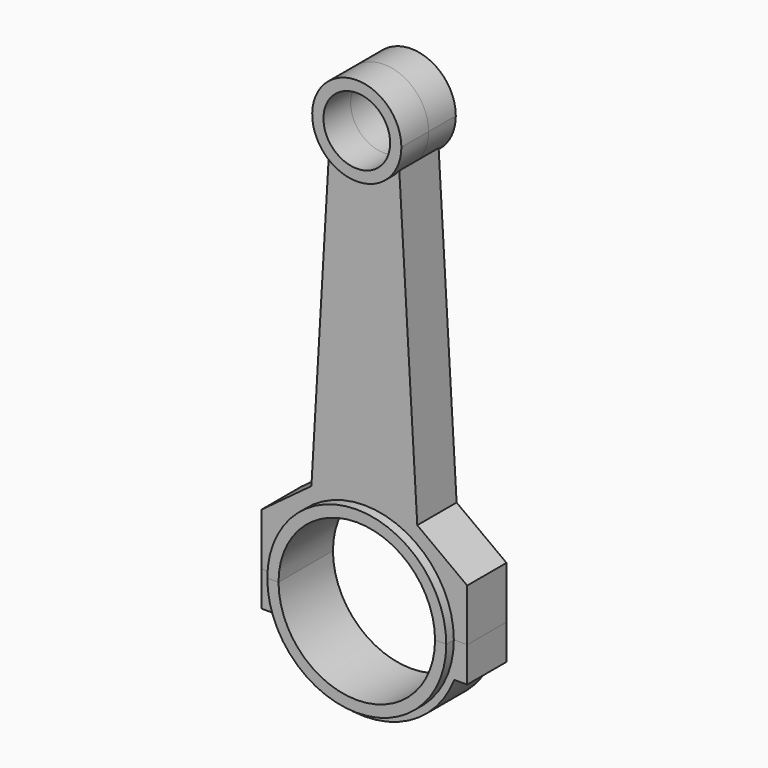
from build123d import *

# Parameters (mm, degrees)
F1_DEPTH = 12.3063
F2_DEPTH = 8.89
F0_R     = 12.065
F3_DEPTH = 12.3063
F4_DEPTH = 12.3063
F5_DEPTH = 8.89


with BuildPart() as f1:
    # F0 (on Front) → F1 (new body, symmetric)
    with BuildSketch(Plane.XZ):
        with BuildLine():
            ThreePointArc((-28.3083, 0), (0, 28.3083), (28.3083, 0))
            Line((28.3083, 0), (32.3723, 0))
            ThreePointArc((32.3723, 0), (0, 32.3723), (-32.3723, 0))
            Line((-32.3723, 0), (-28.3083, 0))
        make_face()
    extrude(amount=F1_DEPTH, both=True)

    # F0 (on Front) → F2 (join, symmetric)
    with BuildSketch(Plane.XZ):
        with BuildLine():
            ThreePointArc((-32.3723, 0), (0, 32.3723), (32.3723, 0))
            Line((32.3723, 0), (37.1983, 0))
            Line((37.1983, 0), (37.1983, 18.8489910215))
            Line((37.1983, 18.8489910215), (19.1531982273, 32.195366919))
            Line((19.1531982273, 32.195366919), (12.6520330329, 142.9806655679))
            ThreePointArc((12.6520330329, 142.9806655679), (0, 136.8552), (-12.6520330329, 142.9806655679))
            Line((-12.6520330329, 142.9806655679), (-19.1531982273, 32.195366919))
            Line((-19.1531982273, 32.195366919), (-37.1983, 18.8489910215))
            Line((-37.1983, 18.8489910215), (-37.1983, 0))
            Line((-37.1983, 0), (-32.3723, 0))
        make_face()
    extrude(amount=F2_DEPTH, both=True)

    # F0 (on Front) → F3 (join, symmetric)
    with BuildSketch(Plane.XZ):
        with BuildLine():
            ThreePointArc((-12.6520330329, 142.9806655679), (0, 136.8552), (12.6520330329, 142.9806655679))
            ThreePointArc((12.6520330329, 142.9806655679), (15.2349808301, 147.6889190721), (16.129, 152.9842))
            ThreePointArc((16.129, 152.9842), (-5.2952809279, 168.2191808301), (-12.6520330329, 142.9806655679))
        make_face()
        with Locations((0, 152.9842)):
            Circle(F0_R, mode=Mode.SUBTRACT)
    extrude(amount=F3_DEPTH, both=True)


with BuildPart() as f4:
    # F0 (on Front) → F4 (new body, symmetric)
    with BuildSketch(Plane.XZ):
        with BuildLine():
            Line((32.3723, 0), (28.3083, 0))
            ThreePointArc((28.3083, 0), (0, -28.3083), (-28.3083, 0))
            Line((-28.3083, 0), (-32.3723, 0))
            ThreePointArc((-32.3723, 0), (0, -32.3723), (32.3723, 0))
        make_face()
    extrude(amount=F4_DEPTH, both=True)

    # F0 (on Front) → F5 (join, symmetric)
    with BuildSketch(Plane.XZ):
        with BuildLine():
            Line((37.1983, 0), (32.3723, 0))
            ThreePointArc((32.3723, 0), (0, -32.3723), (-32.3723, 0))
            Line((-32.3723, 0), (-37.1983, 0))
            Line((-37.1983, 0), (-37.1983, -12.7))
            Line((-37.1983, -12.7), (-32.52043498, -12.7))
            ThreePointArc((-32.52043498, -12.7), (0, -34.9123), (32.52043498, -12.7))
            Line((32.52043498, -12.7), (37.1983, -12.7))
            Line((37.1983, -12.7), (37.1983, 0))
        make_face()
    extrude(amount=F5_DEPTH, both=True)


solid = Compound([f1.part, f4.part])
